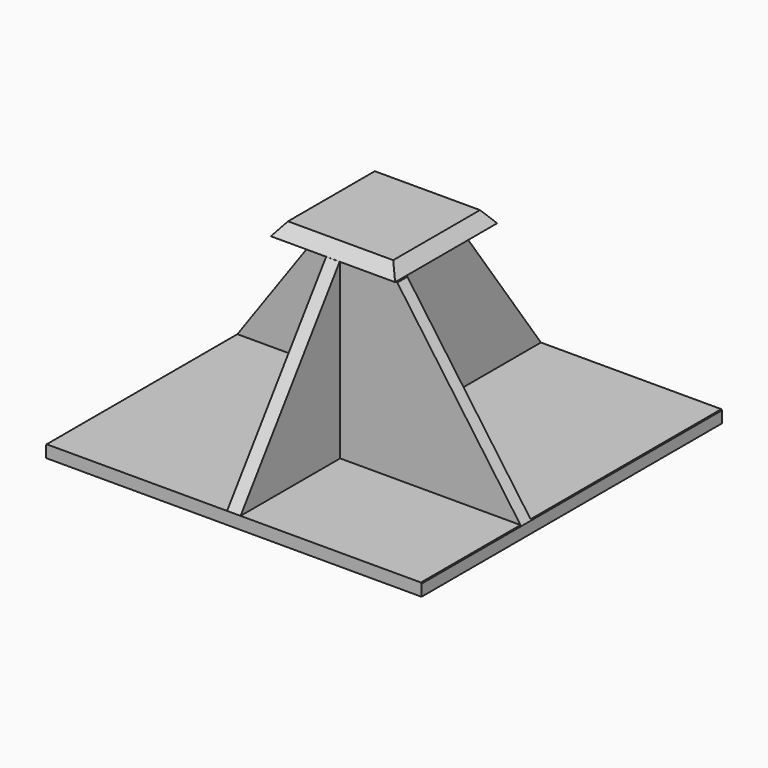
from build123d import *

# Parameters (mm, degrees)
F0_W        = 151.593759656
F0_H        = 151.593759656
F1_DEPTH    = 5
F2_W        = 5.4470277391
F2_H        = 151.593759656
F3_DEPTH    = 70
F4_T1_DEPTH = 366.9308973901
F5_T1_DEPTH = 366.9308973901
F6_W        = 50.1838475466
F6_H        = 51.510296762
F7_DEPTH    = 5
F8_SIZE2    = 4.99999
F8_SIZE     = 3.84999
F9_W        = 73.0733659584
F9_H        = 5.1989573985
F10_DEPTH   = 70
F11_SIZE2   = 70.3308355562
F11_SIZE    = 50
F12_W       = 73.0733659584
F12_H       = 5.0847064704
F13_DEPTH   = 70
F14_SIZE2   = 50
F14_SIZE    = 70.3568348711


# Not quite as in the source:
# - a fillet or chamfer that OpenCascade refuses, or shapes differently, is made with other operations: its cross-section is extruded or revolved along the edge and cut away or added
# - a fillet or chamfer is up to 0.001 mm smaller than in the source, because OpenCascade refuses the exact size


with BuildPart() as f1:
    # F0 (on Top) → F1 (new body)
    with BuildSketch(Plane.XY):
        Rectangle(F0_W, F0_H)
    extrude(amount=F1_DEPTH)

    # F2 (on face) → F3 (join)
    with BuildSketch(Plane.XY.offset(5)):
        Rectangle(F2_W, F2_H)
    extrude(amount=F3_DEPTH)

    # F4: chamfer of 50 x 70 on 1 edges, made by hand

    # F4_s2 → F4_t1 (cut)
    with BuildSketch(Plane.YZ.offset(-183.465448695)):
        Polygon((-75.796879828, 5), (-25.796879828, 75), (-75.796879828, 75), align=None)
    extrude(amount=F4_T1_DEPTH, mode=Mode.SUBTRACT)

    # F5: chamfer of 70 x 50 on 1 edges, made by hand

    # F5_s2 → F5_t1 (cut)
    with BuildSketch(Plane.YZ.offset(-183.465448695)):
        Polygon((75.796879828, 5), (25.796879828, 75), (75.796879828, 75), align=None)
    extrude(amount=F5_T1_DEPTH, mode=Mode.SUBTRACT)

    # F6 (on face) → F7 (join)
    with BuildSketch(Plane.XY.offset(75)):
        Rectangle(F6_W, F6_H)
    extrude(amount=F7_DEPTH)

    # F8 (size 3.85 and 5 in the source; OpenCascade refuses exactly that, so slightly less here)
    f8_edges = [f1.edges().sort_by_distance(p)[0] for p in [
        (25.091924, 0, 80),
        (0, -25.755148, 80),
        (0, 25.755148, 80),
        (-25.091924, 0, 80),
    ]]
    f8_side = f1.faces().sort_by_distance((0, 0, 80))[0]
    chamfer(f8_edges, length=F8_SIZE, length2=F8_SIZE2, reference=f8_side)

    # F9 (on face) → F10 (join)
    with BuildSketch(Plane.XY.offset(5)):
        with Locations((-39.2601968488, 23.0562509969)):
            Rectangle(F9_W, F9_H)
    extrude(amount=F10_DEPTH)

    # F11
    f11_edges = [f1.edges().sort_by_distance(p)[0] for p in [
        (-75.79688, 23.056251, 75),
    ]]
    f11_side = f1.faces().sort_by_distance((-50.444402, 23.056251, 75))[0]
    chamfer(f11_edges, length=F11_SIZE, length2=F11_SIZE2, reference=f11_side)

    # F12 (on face) → F13 (join)
    with BuildSketch(Plane.XY.offset(5)):
        with Locations((39.2601968488, -22.9917196557)):
            Rectangle(F12_W, F12_H)
    extrude(amount=F13_DEPTH)

    # F14
    f14_edges = [f1.edges().sort_by_distance(p)[0] for p in [
        (75.79688, -22.99172, 75),
    ]]
    f14_side = f1.faces().sort_by_distance((75.79688, -74.105559, 2.5))[0]
    chamfer(f14_edges, length=F14_SIZE, length2=F14_SIZE2, reference=f14_side)


solid = f1.part
